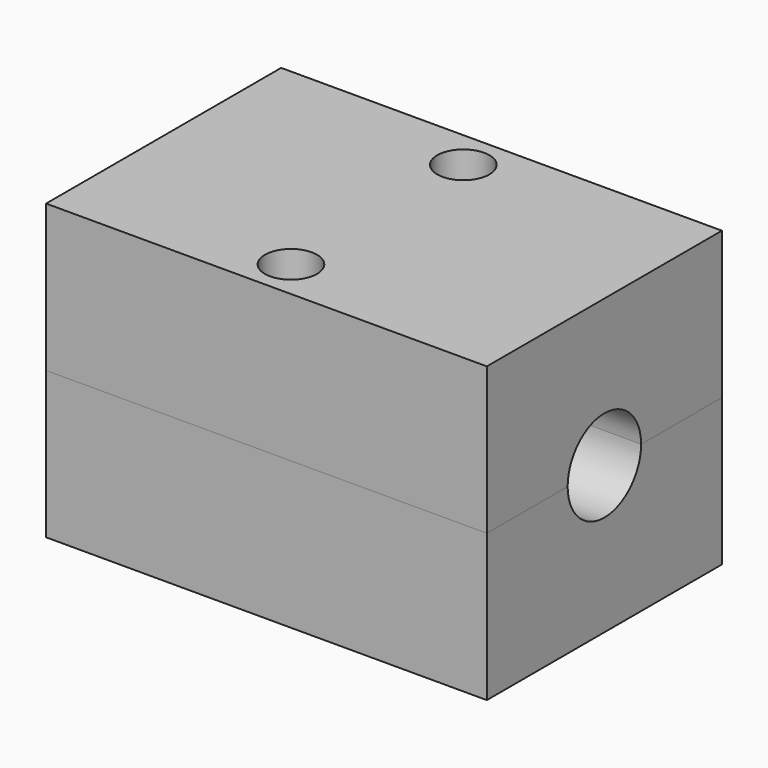
from build123d import *

# Parameters (mm, degrees)
F3_W       = 57.15
F3_H       = 38.1
F4_DEPTH   = 19.05
F5_DEPTH   = 19.05
F7_D       = 11.90752
F7_DEPTH   = 25.4
F7_TIP     = 3.5773799191
F7_2_D     = 11.90752
F7_2_DEPTH = 25.4
F7_2_TIP   = 3.5773799191
F9_D       = 4.699
F9_2_D     = 4.699
F11_D      = 6.7564
F13_D      = 5.1054


# Not quite as in the source:
# - a variable given as a bare number and used for a length is read in inches; the dataset says mm whatever the document's units were


with BuildPart() as f4:
    # F3 (on Top) → F4 (new body)
    with BuildSketch(Plane.XY):
        Rectangle(F3_W, F3_H)
    extrude(amount=F4_DEPTH)

    # F7
    with Locations(Plane.YZ.offset(28.575)):
        with Locations((0, 0)):
            Hole(F7_D / 2, depth=F7_DEPTH)
            with Locations((0, 0, -(F7_DEPTH + F7_TIP / 2))):  # 118° drill point
                Cone(0, F7_D / 2, F7_TIP, mode=Mode.SUBTRACT)

    # F9 (through all)
    with Locations(Plane(origin=(-28.575, 0, 0), x_dir=(0, -1, 0), z_dir=(-1, 0, 0))):
        with Locations((0, 0)):
            Hole(F9_D / 2)

    # F11 (through all)
    with Locations(Plane.XY.offset(19.05)):
        with Locations((-0.889, -13.97), (-0.889, 13.97)):
            Hole(F11_D / 2)


with BuildPart() as f5:
    # F3 (on Top) → F5 (new body)
    with BuildSketch(Plane.XY):
        Rectangle(F3_W, F3_H)
    extrude(amount=-F5_DEPTH)

    # F7#2
    with Locations(Plane.YZ.offset(28.575)):
        with Locations((0, 0)):
            Hole(F7_2_D / 2, depth=F7_2_DEPTH)
            with Locations((0, 0, -(F7_2_DEPTH + F7_2_TIP / 2))):  # 118° drill point
                Cone(0, F7_2_D / 2, F7_2_TIP, mode=Mode.SUBTRACT)

    # F9#2 (through all)
    with Locations(Plane(origin=(-28.575, 0, 0), x_dir=(0, -1, 0), z_dir=(-1, 0, 0))):
        with Locations((0, 0)):
            Hole(F9_2_D / 2)

    # F13 (through all)
    with Locations(Plane.XY):
        with Locations((-0.889, 13.97), (-0.889, -13.97)):
            Hole(F13_D / 2)


solid = Compound([f4.part, f5.part])
